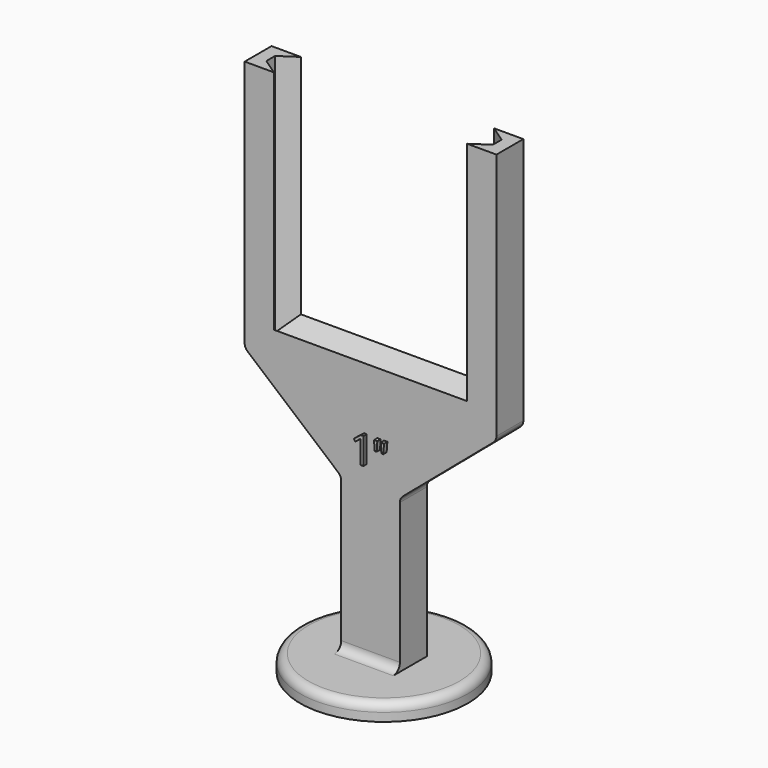
from build123d import *

# Parameters (mm, degrees)
F0_R         = 10
F1_DEPTH     = 2
F2_W         = 7
F2_H         = 28
F3_DEPTH     = 2
F7_TEXT_SIZE = 4.4069547254
F8_DEPTH     = 0.5
F10_DEPTH    = 4
F11_R        = 1


# Not quite as in the source:
# - a feature names something its author has since deleted; it is built from what else it names
# - Text() gives the source's letters only with a copy of the font that has no kerning and outlines rounded to 1/6400 em; it was checked with that copy


with BuildPart() as f1:
    # F0 (on Top) → F1 (new body)
    with BuildSketch(Plane.XY):
        Circle(F0_R)
    extrude(amount=F1_DEPTH)

    # F2 (on Front) → F3 (join, symmetric)
    with BuildSketch(Plane.XZ):
        with Locations((0, 16)):
            Rectangle(F2_W, F2_H)
        Polygon((-15, 30), (-3.5, 30), (3.5, 30), (15, 30), (15, 60), (11.5, 60), (11.5, 33), (-11.5, 33), (-11.5, 60), (-15, 60), align=None)
    extrude(amount=F3_DEPTH, both=True)

    # F6: sweep along a path in F6_path
    with BuildLine(Plane(origin=(-11.5, -2, 60), x_dir=(0, 0, -1), z_dir=(0, 1, 0))) as f6_path:
        Line((0, 0), (27, 0))
        Line((27, 0), (27, -23))
        Line((27, -23), (0, -23))
    # F5 (on face) → F6 (sweep, cut)
    with BuildSketch(Plane.XY.offset(60)):
        Polygon((-11.5, -2), (-11.5, 2), (-13.5, 0.65), (-13.5, -0.65), align=None)
    sweep(path=f6_path.line, transition=Transition.RIGHT, mode=Mode.SUBTRACT)

    # F7 (on face) → F8 (join)
    with BuildSketch(Plane.XZ.offset(2)):
        with Locations((-2, 22.5)):
            Text('1"', F7_TEXT_SIZE, font='Open Sans', text_align=(TextAlign.LEFT, TextAlign.BOTTOM))
    extrude(amount=F8_DEPTH)

    # F9 (on face) → F10 (join)
    with BuildSketch(Plane.XZ.offset(2)):
        Polygon((-3.5, 30), (-15, 30), (-3.5, 20.2310867608), align=None)
        Polygon((3.5, 30), (3.5, 20.2310867608), (15, 30), align=None)
    extrude(amount=-F10_DEPTH)

    # F11
    f11_edges = [f1.edges().sort_by_distance(p)[0] for p in [
        (0, -2, 2),
        (-10, 0, 2),
        (-3.5, 0, 20.231087),
        (-15, 0, 30),
        (15, 0, 30),
        (3.5, 0, 20.231087),
    ]]
    fillet(f11_edges, radius=F11_R)


solid = f1.part
